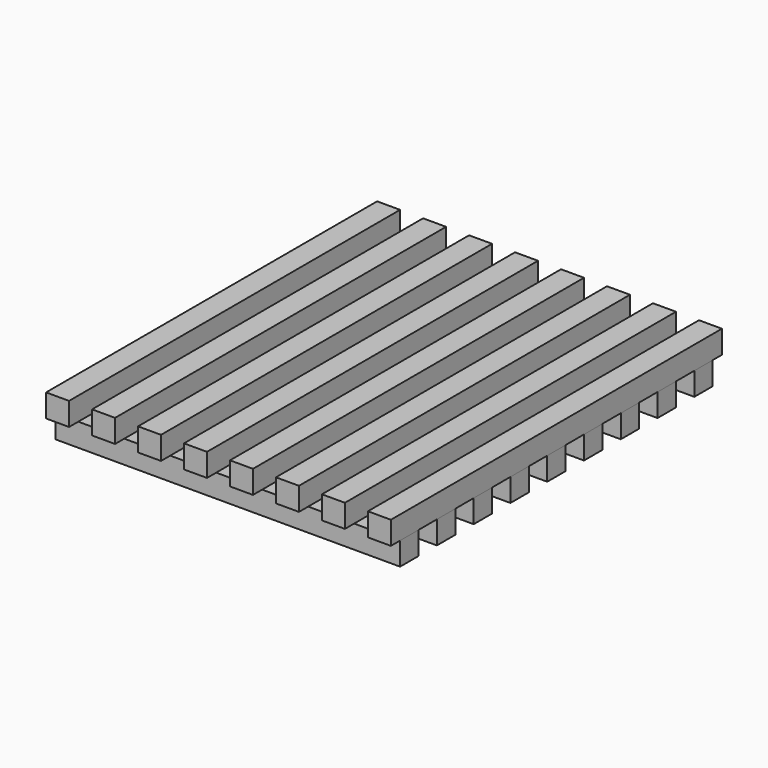
from build123d import *

# Parameters (mm, degrees)
F0_W     = 150
F0_H     = 10
F1_DEPTH = 10
F2_DEPTH = 10
F3_W     = 10
F3_H     = 180
F4_DEPTH = 10


# Not quite as in the source:
# - a feature names something its author has since deleted; it is built from what else it names


with BuildPart() as f1:
    # F0 (on Top) → F1 (new body)
    with BuildSketch(Plane.XY):
        with Locations((0, 50)):
            Rectangle(F0_W, F0_H)
    extrude(amount=F1_DEPTH)


with BuildPart() as f1b:
    # F0 (on Top) → F1, piece 2 (new body)
    with BuildSketch(Plane.XY):
        with Locations((0, 30)):
            Rectangle(F0_W, F0_H)
    extrude(amount=F1_DEPTH)


with BuildPart() as f1c:
    # F0 (on Top) → F1, piece 3 (new body)
    with BuildSketch(Plane.XY):
        with Locations((0, 10)):
            Rectangle(F0_W, F0_H)
    extrude(amount=F1_DEPTH)


with BuildPart() as f1d:
    # F0 (on Top) → F1, piece 4 (new body)
    with BuildSketch(Plane.XY):
        with Locations((0, -10)):
            Rectangle(F0_W, F0_H)
    extrude(amount=F1_DEPTH)


with BuildPart() as f1e:
    # F0 (on Top) → F1, piece 5 (new body)
    with BuildSketch(Plane.XY):
        with Locations((0, -30)):
            Rectangle(F0_W, F0_H)
    extrude(amount=F1_DEPTH)


with BuildPart() as f1f:
    # F0 (on Top) → F1, piece 6 (new body)
    with BuildSketch(Plane.XY):
        with Locations((0, -50)):
            Rectangle(F0_W, F0_H)
    extrude(amount=F1_DEPTH)


with BuildPart() as f1g:
    # F0 (on Top) → F1, piece 7 (new body)
    with BuildSketch(Plane.XY):
        with Locations((0, -70)):
            Rectangle(F0_W, F0_H)
    extrude(amount=F1_DEPTH)


with BuildPart() as f2:
    # F0 (on Top) → F2 (new body)
    with BuildSketch(Plane.XY):
        with Locations((0, 90)):
            Rectangle(F0_W, F0_H)
    extrude(amount=F2_DEPTH)


with BuildPart() as f2b:
    # F0 (on Top) → F2, piece 2 (new body)
    with BuildSketch(Plane.XY):
        with Locations((0, 70)):
            Rectangle(F0_W, F0_H)
    extrude(amount=F2_DEPTH)


with BuildPart() as f2c:
    # F0 (on Top) → F2, piece 3 (new body)
    with BuildSketch(Plane.XY):
        with Locations((0, 50)):
            Rectangle(F0_W, F0_H)
    extrude(amount=F2_DEPTH)


with BuildPart() as f2d:
    # F0 (on Top) → F2, piece 4 (new body)
    with BuildSketch(Plane.XY):
        with Locations((0, 30)):
            Rectangle(F0_W, F0_H)
    extrude(amount=F2_DEPTH)


with BuildPart() as f2e:
    # F0 (on Top) → F2, piece 5 (new body)
    with BuildSketch(Plane.XY):
        with Locations((0, 10)):
            Rectangle(F0_W, F0_H)
    extrude(amount=F2_DEPTH)


with BuildPart() as f2f:
    # F0 (on Top) → F2, piece 6 (new body)
    with BuildSketch(Plane.XY):
        with Locations((0, -10)):
            Rectangle(F0_W, F0_H)
    extrude(amount=F2_DEPTH)


with BuildPart() as f2g:
    # F0 (on Top) → F2, piece 7 (new body)
    with BuildSketch(Plane.XY):
        with Locations((0, -30)):
            Rectangle(F0_W, F0_H)
    extrude(amount=F2_DEPTH)


with BuildPart() as f2h:
    # F0 (on Top) → F2, piece 8 (new body)
    with BuildSketch(Plane.XY):
        with Locations((0, -50)):
            Rectangle(F0_W, F0_H)
    extrude(amount=F2_DEPTH)


with BuildPart() as f2i:
    # F0 (on Top) → F2, piece 9 (new body)
    with BuildSketch(Plane.XY):
        with Locations((0, -70)):
            Rectangle(F0_W, F0_H)
    extrude(amount=F2_DEPTH)


with BuildPart() as f4:
    # F3 (on face) → F4 (new body)
    with BuildSketch(Plane.XY.offset(10)):
        with Locations((70, 10)):
            Rectangle(F3_W, F3_H)
    extrude(amount=F4_DEPTH)


with BuildPart() as f4b:
    # F3 (on face) → F4, piece 2 (new body)
    with BuildSketch(Plane.XY.offset(10)):
        with Locations((50, 10.0000017881)):
            Rectangle(F3_W, F3_H)
    extrude(amount=F4_DEPTH)


with BuildPart() as f4c:
    # F3 (on face) → F4, piece 3 (new body)
    with BuildSketch(Plane.XY.offset(10)):
        with Locations((30, 10.0000017881)):
            Rectangle(F3_W, F3_H)
    extrude(amount=F4_DEPTH)


with BuildPart() as f4d:
    # F3 (on face) → F4, piece 4 (new body)
    with BuildSketch(Plane.XY.offset(10)):
        with Locations((9.9999859929, 10.000000298)):
            Rectangle(F3_W, F3_H)
    extrude(amount=F4_DEPTH)


with BuildPart() as f4e:
    # F3 (on face) → F4, piece 5 (new body)
    with BuildSketch(Plane.XY.offset(10)):
        with Locations((-10, 10.0000017881)):
            Rectangle(F3_W, F3_H)
    extrude(amount=F4_DEPTH)


with BuildPart() as f4f:
    # F3 (on face) → F4, piece 6 (new body)
    with BuildSketch(Plane.XY.offset(10)):
        with Locations((-30, 10.0000017881)):
            Rectangle(F3_W, F3_H)
    extrude(amount=F4_DEPTH)


with BuildPart() as f4g:
    # F3 (on face) → F4, piece 7 (new body)
    with BuildSketch(Plane.XY.offset(10)):
        with Locations((-50, 10.0000017881)):
            Rectangle(F3_W, F3_H)
    extrude(amount=F4_DEPTH)


with BuildPart() as f4h:
    # F3 (on face) → F4, piece 8 (new body)
    with BuildSketch(Plane.XY.offset(10)):
        with Locations((-70, 10.0000017881)):
            Rectangle(F3_W, F3_H)
    extrude(amount=F4_DEPTH)


solid = Compound([f1.part, f1b.part, f1c.part, f1d.part, f1e.part, f1f.part, f1g.part, f2.part, f2b.part, f2c.part, f2d.part, f2e.part, f2f.part, f2g.part, f2h.part, f2i.part, f4.part, f4b.part, f4c.part, f4d.part, f4e.part, f4f.part, f4g.part, f4h.part])
